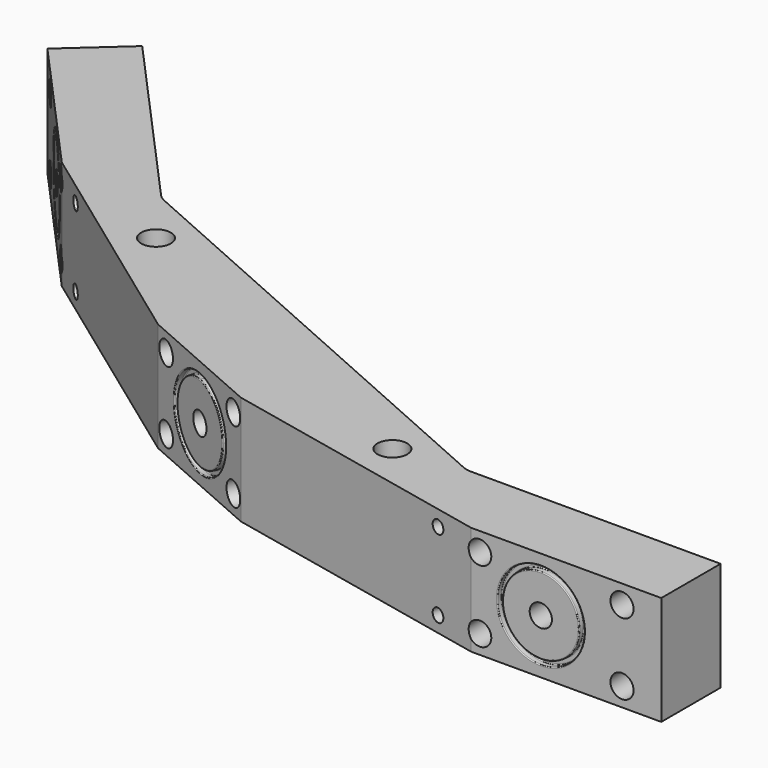
from build123d import *

# Parameters (mm, degrees)
F1_DEPTH  = 25
F3_D      = 5.1054
F5_D      = 5.1054
F7_D      = 5.1054
F9_D      = 3.02
F11_D     = 3.02
F13_D     = 5.3
F15_D     = 5.3
F17_D     = 5.3
F18_R     = 10
F18_R_2   = 8.8
F19_DEPTH = 1.3
F19_TAPER = -2
F20_R     = 0.2
F21_R     = 0.2
F23_DEPTH = 1.3
F23_TAPER = 2
F24_R     = 0.2
F25_R     = 10
F25_R_2   = 8.8
F26_DEPTH = 1.3
F26_TAPER = 2
F27_R     = 0.2
F28_R     = 0.2
F29_R     = 0.2
F30_R     = 0.2
F32_D     = 6.8
F32_DEPTH = 10
F32_TIP   = 2.0429261047
F34_D     = 6.8
F34_DEPTH = 10
F34_TIP   = 2.0429261047


# Not quite as in the source:
# - a feature names something its author has since deleted; it is built from what else it names


with BuildPart() as f1:
    # F0 (on Top) → F1 (new body)
    with BuildSketch(Plane.XY):
        with BuildLine():
            Line((-191.2181864707, -134.3492486113), (-161.703509809, -167.1286178829))
            Line((-161.703509809, -167.1286178829), (-108.9796285159, -205.4347598839))
            Line((-108.9796285159, -205.4347598839), (-79.6950900408, -218.3343625024))
            Line((-79.6950900408, -218.3343625024), (-16, -232))
            Line((-16, -232), (0, -232))
            Line((0, -232), (27.610408524, -232))
            Line((27.610408524, -232), (27.610408524, -215))
            Line((27.610408524, -215), (-16, -215))
            Line((-16, -215), (-29.6074226995, -215))
            ThreePointArc((-29.6074226995, -215), (-30.6452429023, -214.8911071576), (-31.6378586283, -214.5691716907))
            Line((-31.6378586283, -214.5691716907), (-44.4518925955, -208.8749065763))
            Line((-44.4518925955, -208.8749065763), (-125.5675766797, -172.8289423394))
            Line((-125.5675766797, -172.8289423394), (-138.143329782, -167.2405638193))
            ThreePointArc((-138.143329782, -167.2405638193), (-139.0503822914, -166.7175213499), (-139.8286179805, -166.0170451604))
            Line((-139.8286179805, -166.0170451604), (-149.0700477759, -155.7533975748))
            Line((-149.0700477759, -155.7533975748), (-178.5847244376, -122.9740283032))
            Line((-178.5847244376, -122.9740283032), (-191.2181864707, -134.3492486113))
        make_face()
    extrude(amount=F1_DEPTH)

    # F3 (through all)
    with Locations(Plane(origin=(0, -215, 0), x_dir=(-1, 0, 0), z_dir=(0, 1, 0))):
        with Locations((0, 12.5)):
            Hole(F3_D / 2)

    # F5 (through all)
    with Locations(Plane(origin=(-159.7761374776, -143.8630803671, 0), x_dir=(-0.6691306064, 0.7431448255, 0), z_dir=(0.7431448255, 0.6691306064, 0))):
        with Locations((0, 12.5)):
            Hole(F5_D / 2)

    # F7 (through all)
    with Locations(Plane(origin=(-84.8431484065, -190.9259515883, 0), x_dir=(-0.9138343381, 0.4060871858, 0), z_dir=(0.4060871858, 0.9138343381, 0))):
        with Locations((0, 12.5)):
            Hole(F7_D / 2)

    # F9 (through all)
    with Locations(Plane(origin=(-48.2887982282, -225.0725113735, 0), x_dir=(0.9777498949, -0.2097740284, 0), z_dir=(-0.2097740284, -0.9777498949, 0))):
        with Locations((23.6874529505, 21.4171517816), (23.6874529505, 3.5828482184)):
            Hole(F9_D / 2)

    # F11 (through all)
    with Locations(Plane(origin=(-135.3415691624, -186.2816888834, 0), x_dir=(0.8090169944, -0.5877852523, 0), z_dir=(-0.5877852523, -0.8090169944, 0))):
        with Locations((-23.2485540845, 21.4183852211), (-23.2485540845, 3.5816147789)):
            Hole(F11_D / 2)

    # F13 (through all)
    with Locations(Plane(origin=(0, -215, 0), x_dir=(-1, 0, 0), z_dir=(0, 1, 0))):
        with Locations((-18.610408524, 20.7), (-18.610408524, 4.3), (-30.610408524, 20.7), (-30.610408524, 4.3), (13.9985070878, 20.7), (13.9985070878, 4.3)):
            Hole(F13_D / 2)

    # F15 (through all)
    with Locations(Plane(origin=(-159.7761374776, -143.8630803671, 0), x_dir=(-0.6691306064, 0.7431448255, 0), z_dir=(0.7431448255, 0.6691306064, 0))):
        with Locations((19.1089921477, 20.7), (19.1089921477, 4.3), (-13.8510539843, 20.7), (-13.8510539843, 4.3)):
            Hole(F15_D / 2)

    # F17 (through all)
    with Locations(Plane(origin=(-84.8431484065, -190.9259515883, 0), x_dir=(-0.9138343381, 0.4060871858, 0), z_dir=(0.4060871858, 0.9138343381, 0))):
        with Locations((-12.9480805254, 20.7), (13.0519194746, 20.7), (13.0519194746, 4.3), (-12.9480805254, 4.3)):
            Hole(F17_D / 2)

    # F18 (on face) → F19 (cut)
    with BuildSketch(Plane(origin=(-172.4095995108, -155.2383006752, 0), x_dir=(0.6691306064, -0.7431448255, 0), z_dir=(-0.7431448255, -0.6691306064, 0))):
        with Locations((0, 12.5)):
            Circle(F18_R)
        with Locations((0, 12.5)):
            Circle(F18_R_2, mode=Mode.SUBTRACT)
    extrude(amount=-F19_DEPTH, taper=F19_TAPER, mode=Mode.SUBTRACT)

    # F20
    f20_edges = [f1.edges().sort_by_distance(p)[0] for p in [
        (-179.100906, -147.806852, 12.5),
        (-178.165194, -146.903246, 12.5),
    ]]
    fillet(f20_edges, radius=F20_R)

    # F21
    f21_edges = [f1.edges().sort_by_distance(p)[0] for p in [
        (-178.297949, -148.698626, 12.5),
    ]]
    fillet(f21_edges, radius=F21_R)

    # F22 (on face) → F23 (cut)
    with BuildSketch(Plane(origin=(-93.4965770691, -212.2549189639, 0), x_dir=(0.9151490032, -0.4031157427, 0), z_dir=(-0.4031157427, -0.9151490032, 0))):
        with BuildLine():
            ThreePointArc((9.2463759394, 12.5), (6.2705913161, 19.6176118425), (-0.8857037288, 22.49912771))
            ThreePointArc((-0.8857037288, 22.49912771), (-7.7778394374, 5.3823881575), (9.2463759394, 12.5))
        make_face()
        with BuildLine():
            ThreePointArc((8.0463759394, 12.5), (-6.9349335922, 6.2365015786), (-0.8698541686, 21.2992323848))
            ThreePointArc((-0.8698541686, 21.2992323848), (5.4276854709, 18.7634984214), (8.0463759394, 12.5))
        make_face(mode=Mode.SUBTRACT)
    extrude(amount=-F23_DEPTH, taper=F23_TAPER, mode=Mode.SUBTRACT)

    # F24
    f24_edges = [f1.edges().sort_by_distance(p)[0] for p in [
        (-103.337745, -207.919964, 12.5),
        (-94.079888, -211.997975, 3.700768),
        (-102.77215, -206.74857, 12.5),
    ]]
    fillet(f24_edges, radius=F24_R)

    # F25 (on face) → F26 (cut)
    with BuildSketch(Plane.XZ.offset(232)):
        with Locations((0, 12.5)):
            Circle(F25_R)
        with Locations((0, 12.5)):
            Circle(F25_R_2, mode=Mode.SUBTRACT)
    extrude(amount=-F26_DEPTH, taper=F26_TAPER, mode=Mode.SUBTRACT)

    # F27
    f27_edges = [f1.edges().sort_by_distance(p)[0] for p in [
        (-10, -232, 12.5),
        (-9.954603, -230.7, 12.5),
    ]]
    fillet(f27_edges, radius=F27_R)

    # F28
    f28_edges = [f1.edges().sort_by_distance(p)[0] for p in [
        (-8.8, -232, 12.5),
        (-8.845397, -230.7, 12.5),
    ]]
    fillet(f28_edges, radius=F28_R)

    # F29
    f29_edges = [f1.edges().sort_by_distance(p)[0] for p in [
        (-93.555288, -210.808523, 3.655375),
    ]]
    fillet(f29_edges, radius=F29_R)

    # F30
    f30_edges = [f1.edges().sort_by_distance(p)[0] for p in [
        (-177.301484, -147.862493, 12.5),
    ]]
    fillet(f30_edges, radius=F30_R)

    # F32
    with Locations(Plane(origin=(-84.8431484065, -190.9259515883, 0), x_dir=(-0.9138343381, 0.4060871858, 0), z_dir=(0.4060871858, 0.9138343381, 0))):
        with Locations((46.0519194746, 7), (-45.9480805254, 7)):
            Hole(F32_D / 2, depth=F32_DEPTH)
            with Locations((0, 0, -(F32_DEPTH + F32_TIP / 2))):  # 118° drill point
                Cone(0, F32_D / 2, F32_TIP, mode=Mode.SUBTRACT)

    # F34
    with Locations(Plane.XY.offset(25)):
        with Locations((-46.0993034434, -216.8971566265), (-130.1792799391, -179.5339282937)):
            Hole(F34_D / 2, depth=F34_DEPTH)
            with Locations((0, 0, -(F34_DEPTH + F34_TIP / 2))):  # 118° drill point
                Cone(0, F34_D / 2, F34_TIP, mode=Mode.SUBTRACT)


solid = f1.part
